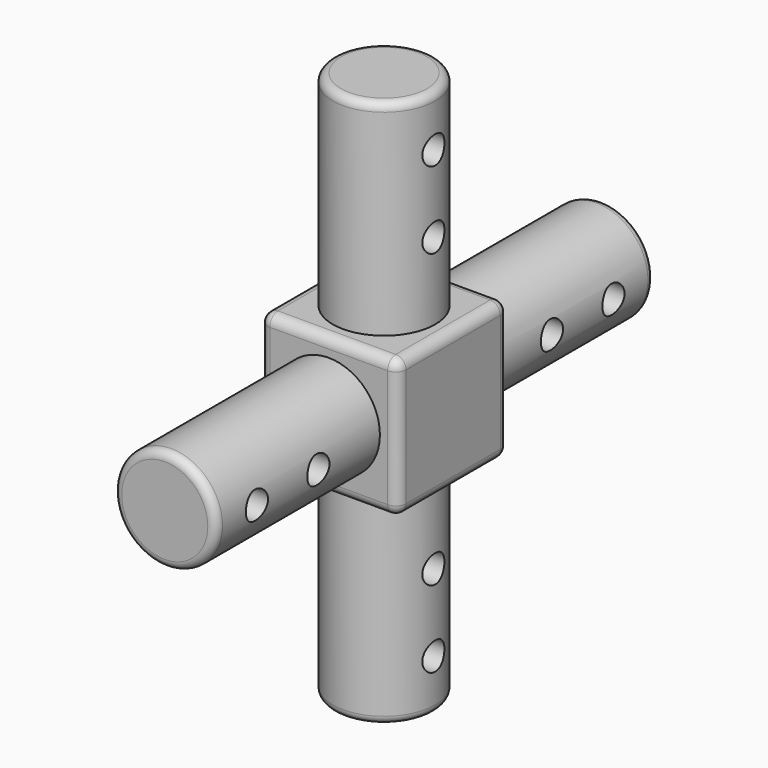
from build123d import *

# Parameters (mm, degrees)
F0_W      = 34.29
F0_H      = 34.29
F1_DEPTH  = 34.29
F2_R      = 12.7
F3_DEPTH  = 50.8
F4_R      = 12.7
F5_DEPTH  = 50.8
F6_R      = 3.429
F7_DEPTH  = 25.4
F8_R      = 3.429
F9_DEPTH  = 25.4
F10_R     = 3.429
F11_DEPTH = 25.4
F12_R     = 2.54
F13_R     = 12.7
F14_DEPTH = 50.8
F15_R     = 3.429
F16_DEPTH = 25.4
F17_R     = 3.429
F18_DEPTH = 25.4
F19_R     = 12.7
F20_DEPTH = 50.8
F21_R     = 3.429
F22_DEPTH = 25.4
F23_R     = 2.032


with BuildPart() as f1:
    # F0 (on Top) → F1 (new body)
    with BuildSketch(Plane.XY):
        with Locations((3.6728888822, 6.5610635031)):
            Rectangle(F0_W, F0_H)
    extrude(amount=F1_DEPTH)

    # F2 (on face) → F3 (join)
    with BuildSketch(Plane.XY.offset(34.29)):
        with Locations((3.6828479417, 6.5610635031)):
            Circle(F2_R)
    extrude(amount=F3_DEPTH)

    # F4 (on face) → F5 (join)
    with BuildSketch(Plane.XZ.offset(10.5839364969)):
        with Locations((3.6728888822, 17.145)):
            Circle(F4_R)
    extrude(amount=F5_DEPTH)

    # F6 (on Right) → F7 (cut, symmetric)
    with BuildSketch(Plane.YZ):
        with Locations((6.5610635031, 53.34)):
            Circle(F6_R)
        with Locations((6.5610635031, 72.39)):
            Circle(F6_R)
    extrude(amount=F7_DEPTH, both=True, mode=Mode.SUBTRACT)

    # F8 (on Right) → F9 (cut, symmetric)
    with BuildSketch(Plane.YZ):
        with Locations((-29.6339364969, 17.145)):
            Circle(F8_R)
        with Locations((-48.6839364969, 17.145)):
            Circle(F8_R)
    extrude(amount=F9_DEPTH, both=True, mode=Mode.SUBTRACT)

    # F10 (on Front) → F11 (cut, symmetric)
    with BuildSketch(Plane.XZ):
        with Locations((-51.5721111178, 17.145)):
            Circle(F10_R)
        with Locations((-32.5221111178, 17.145)):
            Circle(F10_R)
    extrude(amount=F11_DEPTH, both=True, mode=Mode.SUBTRACT)

    # F12
    f12_edges = [f1.edges().sort_by_distance(p)[0] for p in [
        (20.817889, 23.706064, 17.145),
        (20.817889, 6.561064, 34.29),
        (20.817889, -10.583936, 17.145),
        (20.817889, 6.561064, 0),
        (3.672889, 23.706064, 0),
        (3.672889, 23.706064, 34.29),
        (-13.472111, 23.706064, 17.145),
        (-13.472111, 6.561064, 0),
        (3.672889, -10.583936, 0),
        (-13.472111, 6.561064, 34.29),
        (-13.472111, -10.583936, 17.145),
        (3.672889, -10.583936, 34.29),
    ]]
    fillet(f12_edges, radius=F12_R)

    # F13 (on face) → F14 (join)
    with BuildSketch(Plane(origin=(0, 23.7060635031, 0), x_dir=(-1, 0, 0), z_dir=(0, 1, 0))):
        with Locations((-3.6728888822, 17.145)):
            Circle(F13_R)
    extrude(amount=F14_DEPTH)

    # F15 (on Right) → F16 (cut, symmetric)
    with BuildSketch(Plane.YZ):
        with Locations((42.7560635031, 17.145)):
            Circle(F15_R)
        with Locations((61.8060635031, 17.145)):
            Circle(F15_R)
    extrude(amount=F16_DEPTH, both=True, mode=Mode.SUBTRACT)

    # F17 (on Front) → F18 (cut, symmetric)
    with BuildSketch(Plane.XZ):
        with Locations((58.9178888822, 17.145)):
            Circle(F17_R)
        with Locations((39.8678888822, 17.145)):
            Circle(F17_R)
    extrude(amount=F18_DEPTH, both=True, mode=Mode.SUBTRACT)

    # F19 (on face) → F20 (join)
    with BuildSketch(Plane(origin=(0, 0, 0), x_dir=(1, 0, 0), z_dir=(0, 0, -1))):
        with Locations((3.6728888822, -6.5610635031)):
            Circle(F19_R)
    extrude(amount=F20_DEPTH)

    # F21 (on Right) → F22 (cut, symmetric)
    with BuildSketch(Plane.YZ):
        with Locations((6.5610635031, -19.05)):
            Circle(F21_R)
        with Locations((6.5610635031, -38.1)):
            Circle(F21_R)
    extrude(amount=F22_DEPTH, both=True, mode=Mode.SUBTRACT)

    # F23
    f23_edges = [f1.edges().sort_by_distance(p)[0] for p in [
        (-9.017152, 6.561064, 85.09),
        (-9.027111, -61.383936, 17.145),
        (16.372889, 74.506064, 17.145),
        (-9.027111, 6.561064, -50.8),
    ]]
    fillet(f23_edges, radius=F23_R)


solid = f1.part
